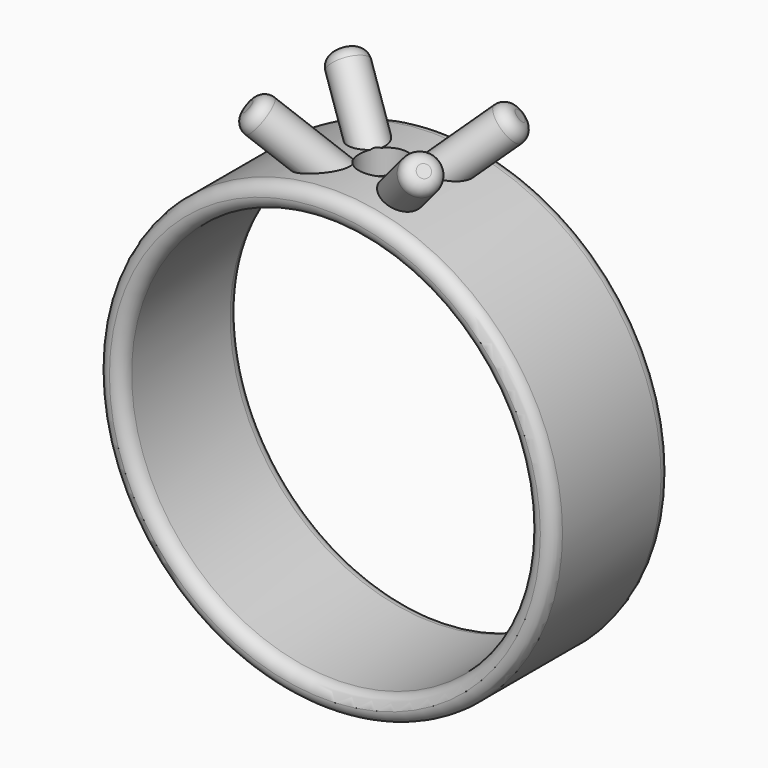
from build123d import *

# Parameters (mm, degrees)
F0_R      = 9.25
F0_R_2    = 8.25
F1_DEPTH  = 3
F10_R     = 0.75
F11_R     = 0.75
F15_R     = 1
F16_DEPTH = 9
F18_R     = 8.25
F19_DEPTH = 25
F20_R     = 0.49999


# Not quite as in the source:
# - a fillet or chamfer is up to 0.001 mm smaller than in the source, because OpenCascade refuses the exact size


with BuildPart() as f1:
    # F0 (on Front) → F1 (new body)
    with BuildSketch(Plane.XZ):
        Circle(F0_R)
        Circle(F0_R_2, mode=Mode.SUBTRACT)
    extrude(amount=F1_DEPTH)

    # F12: sweep along a path in F6
    with BuildLine(Plane(origin=(-3.7456595483, 0, 3.7456595483), x_dir=(0, 1, 0), z_dir=(0.7071067812, 0, -0.7071067812))) as f12_path:
        Line((-0.75, 6.7213760956), (-2.440473047, 10.3466072437))
    # F10 (on line) → F12 (sweep)
    with BuildSketch(Plane(origin=(6.67041722, -4.3988640974, 6.67041722), x_dir=(0.7676607959, 0.3528089641, -0.5349978853), z_dir=(0.6408563821, -0.4226182617, 0.6408563821))):
        with Locations((-4.0381385118, 4.052483348)):
            Circle(F10_R)
    sweep(path=f12_path.line)

    # F13: sweep along a path in F7
    with BuildLine(Plane(origin=(3.7456595483, 0, 3.7456595483), x_dir=(0.7071067812, 0, -0.7071067812), z_dir=(-0.7071067812, 0, -0.7071067812))) as f13_path:
        Line((-6.7113760956, 0.76), (-10.3366072437, 2.450473047))
    # F11 (on line) → F13 (sweep)
    with BuildSketch(Plane(origin=(-6.6673174648, -4.3968199371, 6.6673174648), x_dir=(0.2988362387, -0.906307787, -0.2988362387), z_dir=(-0.6408563821, -0.4226182617, 0.6408563821))):
        with Locations((-2.1475561813, 5.2971625332)):
            Circle(F11_R)
    sweep(path=f13_path.line)

    # F15 (on offset) → F16 (cut)
    with BuildSketch(Plane.XY.offset(13)):
        Circle(F15_R)
    extrude(amount=-F16_DEPTH, mode=Mode.SUBTRACT)

    # F17: F1 across face


with BuildPart() as f1_1:
    add(f1.part)
    add(f1.part.mirror(Plane(origin=(0, 0, -0.3303539974), x_dir=(1, 0, 0), z_dir=(0, 1, 0))))

    # F18 (on face) → F19 (cut)
    with BuildSketch(Plane.XZ.offset(3)):
        Circle(F18_R)
    extrude(amount=-F19_DEPTH, mode=Mode.SUBTRACT)

    # F20 (radius 0.5 in the source; OpenCascade refuses exactly that, so slightly less here)
    f20_edges = [f1_1.edges().sort_by_distance(p)[0] for p in [
        (-9.25, -3, 0),
        (-8.25, -3, 0),
        (-9.25, 3, 0),
        (-8.25, 3, 0),
        (2.994751, 2.70508, 11.463064),
        (2.994751, -2.70508, 11.463064),
        (-3.787553, -1.770742, 11.278872),
        (-3.787553, 1.770742, 11.278872),
    ]]
    fillet(f20_edges, radius=F20_R)


solid = f1_1.part
